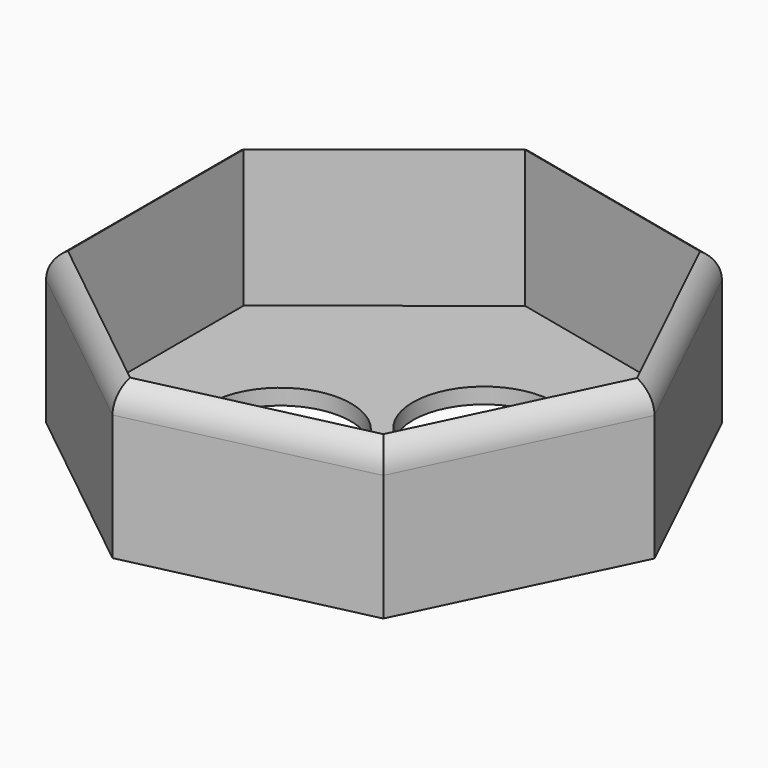
from build123d import *

# Parameters (mm, degrees)
F1_DEPTH     = 25.4
F2_T         = -2.54
F4_D         = 22.86
F6_D         = 22.86
F9_T1_DEPTH  = 63.2859311747
F9_T3_DEPTH  = 63.2859311747
F9_T5_DEPTH  = 63.2859311747
F9_T7_DEPTH  = 63.2859311747
F9_T9_DEPTH  = 63.2859311747
F9_T11_DEPTH = 63.2859311747
F9_T13_DEPTH = 63.2859311747


# Not quite as in the source:
# - a fillet or chamfer that OpenCascade refuses, or shapes differently, is made with other operations: its cross-section is extruded or revolved along the edge and cut away or added
# - the program builds the solid bodies; features that only make, move or delete a surface that nothing else refers to are left out


with BuildPart() as f1:
    # F0 (on Top) → F1 (new body)
    with BuildSketch(Plane.XY):
        Polygon((27.2259101757, 34.1301219533), (-9.7089265027, 42.5658566882), (-39.3327434985, 18.9486331517), (-39.3382023982, -18.9372976297), (-9.721192539, -42.5630570455), (27.2160735783, -34.1379663779), (43.6590811844, -0.0062907401), align=None)
    extrude(amount=F1_DEPTH)

    # F2
    f2_openings = [f1.faces().sort_by_distance(p)[0] for p in [
        (0, 0, 25.4),
    ]]
    offset(amount=F2_T, openings=f2_openings)

    # F4 (through all)
    with Locations(Plane.XY.offset(2.54)):
        with Locations((-12.0702767901, -5.8105965731)):
            Hole(F4_D / 2)

    # F6 (through all)
    with Locations(Plane.XY.offset(2.54)):
        with Locations((7.7538759853, 10.4717538884)):
            Hole(F6_D / 2)

    # F9: fillet of radius 5.08 on 7 edges, made by hand

    # F9_s2 → F9_t1 (cut)
    with BuildSketch(Plane(origin=(30.848595501, -7.0456672344, 0), x_dir=(0, 0, 1), z_dir=(-0.9748958395, 0.2226614068, 0))):
        with BuildLine():
            ThreePointArc((25.4, 34.2554733567), (23.9121024484, 37.8475758051), (20.32, 39.3354733567))
            Line((20.32, 39.3354733567), (25.4, 39.3354733567))
            Line((25.4, 39.3354733567), (25.4, 34.2554733567))
        make_face()
    extrude(amount=F9_T1_DEPTH, mode=Mode.SUBTRACT)

    # F9_s4 → F9_t3 (cut)
    with BuildSketch(Plane(origin=(24.7423091554, 19.7255014847, 0), x_dir=(0, 0, 1), z_dir=(-0.7819213116, -0.623377143, 0))):
        with BuildLine():
            ThreePointArc((25.4, 34.2554733567), (23.9121024484, 37.8475758051), (20.32, 39.3354733567))
            Line((20.32, 39.3354733567), (25.4, 39.3354733567))
            Line((25.4, 39.3354733567), (25.4, 34.2554733567))
        make_face()
    extrude(amount=F9_T3_DEPTH, mode=Mode.SUBTRACT)

    # F9_s6 → F9_t5 (cut)
    with BuildSketch(Plane(origin=(0.0045593646, 31.6429652589, 0), x_dir=(0, 0, 1), z_dir=(-0.0001440878, -0.9999999896, 0))):
        with BuildLine():
            ThreePointArc((25.4, 34.2554733567), (23.9121024484, 37.8475758051), (20.32, 39.3354733567))
            Line((20.32, 39.3354733567), (25.4, 39.3354733567))
            Line((25.4, 39.3354733567), (25.4, 34.2554733567))
        make_face()
    extrude(amount=F9_T5_DEPTH, mode=Mode.SUBTRACT)

    # F9_s8 → F9_t7 (cut)
    with BuildSketch(Plane(origin=(-24.7366237207, 19.7326307943, 0), x_dir=(0, 0, 1), z_dir=(0.7817416371, -0.6236024477, 0))):
        with BuildLine():
            ThreePointArc((25.4, 34.2554733567), (23.9121024484, 37.8475758051), (20.32, 39.3354733567))
            Line((20.32, 39.3354733567), (25.4, 39.3354733567))
            Line((25.4, 39.3354733567), (25.4, 34.2554733567))
        make_face()
    extrude(amount=F9_T7_DEPTH, mode=Mode.SUBTRACT)

    # F9_s10 → F9_t9 (cut)
    with BuildSketch(Plane(origin=(-30.8506246092, -7.0367771307, 0), x_dir=(0, 0, 1), z_dir=(0.9749599646, 0.2223804564, 0))):
        with BuildLine():
            ThreePointArc((20.32, 39.3354733567), (23.9121024484, 37.8475758051), (25.4, 34.2554733567))
            Line((25.4, 34.2554733567), (25.4, 39.3354733567))
            Line((25.4, 39.3354733567), (20.32, 39.3354733567))
        make_face()
    extrude(amount=F9_T9_DEPTH, mode=Mode.SUBTRACT)

    # F9_s12 → F9_t11 (cut)
    with BuildSketch(Plane(origin=(-13.7334759289, -28.5073483522, 0), x_dir=(0, 0, 1), z_dir=(0.4340135532, 0.9009063412, 0))):
        with BuildLine():
            ThreePointArc((20.32, 39.3354733567), (23.9121024484, 37.8475758051), (25.4, 34.2554733567))
            Line((25.4, 34.2554733567), (25.4, 39.3354733567))
            Line((25.4, 39.3354733567), (20.32, 39.3354733567))
        make_face()
    extrude(amount=F9_T11_DEPTH, mode=Mode.SUBTRACT)

    # F9_s14 → F9_t13 (cut)
    with BuildSketch(Plane(origin=(13.7252602377, -28.5113048206, 0), x_dir=(0, 0, 1), z_dir=(-0.433753916, 0.9010313759, 0))):
        with BuildLine():
            ThreePointArc((20.32, 39.3354733567), (23.9121024484, 37.8475758051), (25.4, 34.2554733567))
            Line((25.4, 34.2554733567), (25.4, 39.3354733567))
            Line((25.4, 39.3354733567), (20.32, 39.3354733567))
        make_face()
    extrude(amount=F9_T13_DEPTH, mode=Mode.SUBTRACT)


solid = f1.part
